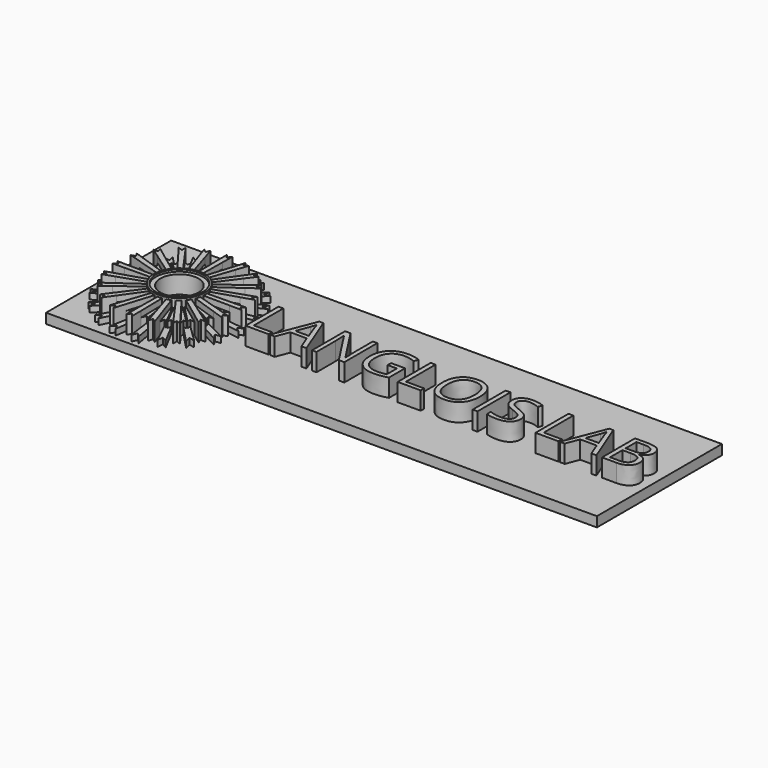
from build123d import *

# Parameters (mm, degrees)
F0_R         = 11.7672405149
F0_R_2       = 9.5549207282
F1_DEPTH     = 9
F2_DEPTH     = 10
F3_DEPTH     = 3
F4_DEPTH     = 6
F5_DEPTH     = 9
F6_TEXT_SIZE = 28.9957211175
F7_DEPTH     = 9
F9_W         = 276.4481753111
F9_H         = 78.4506313503
F10_DEPTH    = 5


# Not quite as in the source:
# - Text() gives the source's letters only with a copy of the font that has no kerning and outlines rounded to 1/6400 em; it was checked with that copy


with BuildPart() as f1:
    # F0 (on Top) → F1 (new body)
    with BuildSketch(Plane.XY):
        Circle(F0_R)
        Circle(F0_R_2, mode=Mode.SUBTRACT)
    extrude(amount=F1_DEPTH)

    # F0 (on Top) → F2 (join)
    with BuildSketch(Plane.XY):
        with BuildLine():
            ThreePointArc((12.7135907926, -0.7743630538), (12.7312599796, -0.3873606999), (12.7371515254, 0))
            ThreePointArc((12.7371515254, 0), (12.715744973, 0.7381454891), (12.6515972691, 1.4738098661))
            ThreePointArc((12.6515972691, 1.4738098661), (12.6226522142, 1.7040187972), (12.589518622, 1.9336622889))
            ThreePointArc((12.589518622, 1.9336622889), (12.5328289853, 2.2722734447), (12.4670336703, 2.609233689))
            ThreePointArc((12.4670336703, 2.609233689), (12.4022605626, 2.901544747), (12.3306347123, 3.1922525861))
            ThreePointArc((12.3306347123, 3.1922525861), (12.0006538998, 4.268411292), (11.5769517292, 5.311235039))
            ThreePointArc((11.5769517292, 5.311235039), (11.4782848741, 5.5212322293), (11.3758092138, 5.7293973254))
            ThreePointArc((11.3758092138, 5.7293973254), (11.2172575638, 6.0339176104), (11.0505560588, 6.334053976))
            ThreePointArc((11.0505560588, 6.334053976), (10.8986240881, 6.5920423215), (10.7406701937, 6.8463883012))
            ThreePointArc((10.7406701937, 6.8463883012), (10.094288463, 7.7679063721), (9.3690734927, 8.6287595208))
            ThreePointArc((9.3690734927, 8.6287595208), (9.2103430367, 8.797988982), (9.0485563398, 8.9642990326))
            ThreePointArc((9.0485563398, 8.9642990326), (8.8036628167, 9.2049198796), (8.5523730266, 9.4388529279))
            ThreePointArc((8.5523730266, 9.4388529279), (8.3281543526, 9.637264864), (8.0993340419, 9.8303518278))
            ThreePointArc((8.0993340419, 9.8303518278), (7.1998237404, 10.5070246544), (6.2440850646, 11.1016409006))
            ThreePointArc((6.2440850646, 11.1016409006), (6.0408286506, 11.213537274), (5.8355677263, 11.3217126925))
            ThreePointArc((5.8355677263, 11.3217126925), (5.5283042144, 11.4748804566), (5.2170241346, 11.6197111909))
            ThreePointArc((5.2170241346, 11.6197111909), (4.9424668435, 11.739124775), (4.6651786428, 11.8520520254))
            ThreePointArc((4.6651786428, 11.8520520254), (3.600590106, 12.2176421567), (2.5078820852, 12.4878163194))
            ThreePointArc((2.5078820852, 12.4878163194), (2.2799958672, 12.5314264083), (2.051353085, 12.5708782311))
            ThreePointArc((2.051353085, 12.5708782311), (1.7117966777, 12.6215997843), (1.3709965711, 12.6631511632))
            ThreePointArc((1.3709965711, 12.6631511632), (1.0729762435, 12.6918773616), (0.7743630538, 12.7135907926))
            ThreePointArc((0.7743630538, 12.7135907926), (-0.3510943748, 12.7323117194), (-1.4738098661, 12.6515972691))
            ThreePointArc((-1.4738098661, 12.6515972691), (-1.7040187972, 12.6226522142), (-1.9336622889, 12.589518622))
            ThreePointArc((-1.9336622889, 12.589518622), (-2.2722734447, 12.5328289853), (-2.609233689, 12.4670336703))
            ThreePointArc((-2.609233689, 12.4670336703), (-2.901544747, 12.4022605626), (-3.1922525861, 12.3306347123))
            ThreePointArc((-3.1922525861, 12.3306347123), (-4.268411292, 12.0006538998), (-5.311235039, 11.5769517292))
            ThreePointArc((-5.311235039, 11.5769517292), (-5.5212322293, 11.4782848741), (-5.7293973254, 11.3758092138))
            ThreePointArc((-5.7293973254, 11.3758092138), (-6.0339176104, 11.2172575638), (-6.334053976, 11.0505560588))
            ThreePointArc((-6.334053976, 11.0505560588), (-6.5920423215, 10.8986240881), (-6.8463883012, 10.7406701937))
            ThreePointArc((-6.8463883012, 10.7406701937), (-7.7679063721, 10.094288463), (-8.6287595208, 9.3690734927))
            ThreePointArc((-8.6287595208, 9.3690734927), (-8.797988982, 9.2103430367), (-8.9642990326, 9.0485563398))
            ThreePointArc((-8.9642990326, 9.0485563398), (-9.2049198796, 8.8036628167), (-9.4388529279, 8.5523730266))
            ThreePointArc((-9.4388529279, 8.5523730266), (-9.637264864, 8.3281543526), (-9.8303518278, 8.0993340419))
            ThreePointArc((-9.8303518278, 8.0993340419), (-10.5070246544, 7.1998237404), (-11.1016409006, 6.2440850646))
            ThreePointArc((-11.1016409006, 6.2440850646), (-11.213537274, 6.0408286506), (-11.3217126925, 5.8355677263))
            ThreePointArc((-11.3217126925, 5.8355677263), (-11.4748804566, 5.5283042144), (-11.6197111909, 5.2170241346))
            ThreePointArc((-11.6197111909, 5.2170241346), (-11.739124775, 4.9424668435), (-11.8520520254, 4.6651786428))
            ThreePointArc((-11.8520520254, 4.6651786428), (-12.2176421567, 3.600590106), (-12.4878163194, 2.5078820852))
            ThreePointArc((-12.4878163194, 2.5078820852), (-12.5314264083, 2.2799958672), (-12.5708782311, 2.051353085))
            ThreePointArc((-12.5708782311, 2.051353085), (-12.6215997843, 1.7117966777), (-12.6631511632, 1.3709965711))
            ThreePointArc((-12.6631511632, 1.3709965711), (-12.6918773616, 1.0729762435), (-12.7135907926, 0.7743630538))
            ThreePointArc((-12.7135907926, 0.7743630538), (-12.7323117194, -0.3510943748), (-12.6515972691, -1.4738098661))
            ThreePointArc((-12.6515972691, -1.4738098661), (-12.6226522142, -1.7040187972), (-12.589518622, -1.9336622889))
            ThreePointArc((-12.589518622, -1.9336622889), (-12.5328289853, -2.2722734447), (-12.4670336703, -2.609233689))
            ThreePointArc((-12.4670336703, -2.609233689), (-12.4022605626, -2.901544747), (-12.3306347123, -3.1922525861))
            ThreePointArc((-12.3306347123, -3.1922525861), (-12.0006538998, -4.268411292), (-11.5769517292, -5.311235039))
            ThreePointArc((-11.5769517292, -5.311235039), (-11.4782848741, -5.5212322293), (-11.3758092138, -5.7293973254))
            ThreePointArc((-11.3758092138, -5.7293973254), (-11.2172575638, -6.0339176104), (-11.0505560588, -6.334053976))
            ThreePointArc((-11.0505560588, -6.334053976), (-10.8986240881, -6.5920423215), (-10.7406701937, -6.8463883012))
            ThreePointArc((-10.7406701937, -6.8463883012), (-10.094288463, -7.7679063721), (-9.3690734927, -8.6287595208))
            ThreePointArc((-9.3690734927, -8.6287595208), (-9.2103430367, -8.797988982), (-9.0485563398, -8.9642990326))
            ThreePointArc((-9.0485563398, -8.9642990326), (-8.8036628167, -9.2049198796), (-8.5523730266, -9.4388529279))
            ThreePointArc((-8.5523730266, -9.4388529279), (-8.3281543526, -9.637264864), (-8.0993340419, -9.8303518278))
            ThreePointArc((-8.0993340419, -9.8303518278), (-7.1998237404, -10.5070246544), (-6.2440850646, -11.1016409006))
            ThreePointArc((-6.2440850646, -11.1016409006), (-6.0408286506, -11.213537274), (-5.8355677263, -11.3217126925))
            ThreePointArc((-5.8355677263, -11.3217126925), (-5.5283042144, -11.4748804566), (-5.2170241346, -11.6197111909))
            ThreePointArc((-5.2170241346, -11.6197111909), (-4.9424668435, -11.739124775), (-4.6651786428, -11.8520520254))
            ThreePointArc((-4.6651786428, -11.8520520254), (-3.600590106, -12.2176421567), (-2.5078820852, -12.4878163194))
            ThreePointArc((-2.5078820852, -12.4878163194), (-2.2799958672, -12.5314264083), (-2.051353085, -12.5708782311))
            ThreePointArc((-2.051353085, -12.5708782311), (-1.7117966777, -12.6215997843), (-1.3709965711, -12.6631511632))
            ThreePointArc((-1.3709965711, -12.6631511632), (-1.0729762435, -12.6918773616), (-0.7743630538, -12.7135907926))
            ThreePointArc((-0.7743630538, -12.7135907926), (0.3510943748, -12.7323117194), (1.4738098661, -12.6515972691))
            ThreePointArc((1.4738098661, -12.6515972691), (1.7040187972, -12.6226522142), (1.9336622889, -12.589518622))
            ThreePointArc((1.9336622889, -12.589518622), (2.2722734447, -12.5328289853), (2.609233689, -12.4670336703))
            ThreePointArc((2.609233689, -12.4670336703), (2.901544747, -12.4022605626), (3.1922525861, -12.3306347123))
            ThreePointArc((3.1922525861, -12.3306347123), (4.268411292, -12.0006538998), (5.311235039, -11.5769517292))
            ThreePointArc((5.311235039, -11.5769517292), (5.5212322293, -11.4782848741), (5.7293973254, -11.3758092138))
            ThreePointArc((5.7293973254, -11.3758092138), (6.0339176104, -11.2172575638), (6.334053976, -11.0505560588))
            ThreePointArc((6.334053976, -11.0505560588), (6.5920423215, -10.8986240881), (6.8463883012, -10.7406701937))
            ThreePointArc((6.8463883012, -10.7406701937), (7.7679063721, -10.094288463), (8.6287595208, -9.3690734927))
            ThreePointArc((8.6287595208, -9.3690734927), (8.797988982, -9.2103430367), (8.9642990326, -9.0485563398))
            ThreePointArc((8.9642990326, -9.0485563398), (9.2049198796, -8.8036628167), (9.4388529279, -8.5523730266))
            ThreePointArc((9.4388529279, -8.5523730266), (9.637264864, -8.3281543526), (9.8303518278, -8.0993340419))
            ThreePointArc((9.8303518278, -8.0993340419), (10.5070246544, -7.1998237404), (11.1016409006, -6.2440850646))
            ThreePointArc((11.1016409006, -6.2440850646), (11.213537274, -6.0408286506), (11.3217126925, -5.8355677263))
            ThreePointArc((11.3217126925, -5.8355677263), (11.4748804566, -5.5283042144), (11.6197111909, -5.2170241346))
            ThreePointArc((11.6197111909, -5.2170241346), (11.739124775, -4.9424668435), (11.8520520254, -4.6651786428))
            ThreePointArc((11.8520520254, -4.6651786428), (12.2176421567, -3.600590106), (12.4878163194, -2.5078820852))
            ThreePointArc((12.4878163194, -2.5078820852), (12.5314264083, -2.2799958672), (12.5708782311, -2.051353085))
            ThreePointArc((12.5708782311, -2.051353085), (12.6215997843, -1.7117966777), (12.6631511632, -1.3709965711))
            ThreePointArc((12.6631511632, -1.3709965711), (12.6918773616, -1.0729762435), (12.7135907926, -0.7743630538))
        make_face()
        Circle(F0_R, mode=Mode.SUBTRACT)
    extrude(amount=F2_DEPTH)

    # F0 (on Top) → F3 (join)
    with BuildSketch(Plane.XY):
        with BuildLine():
            Line((11.6859453374, -21.9507384227), (6.334053976, -11.0505560588))
            ThreePointArc((6.334053976, -11.0505560588), (6.0339176104, -11.2172575638), (5.7293973254, -11.3758092138))
            Line((5.7293973254, -11.3758092138), (11.2666978089, -22.2109639059))
            Line((11.2666978089, -22.2109639059), (9.8357876585, -21.7249978341))
            Line((9.8357876585, -21.7249978341), (15.0472962032, -32.4688493698))
            Line((15.0472962032, -32.4688493698), (15.3143611387, -29.4471931073))
            Line((15.3143611387, -29.4471931073), (17.853469935, -30.9337573252))
            Line((17.853469935, -30.9337573252), (12.2699130015, -20.3598729012))
            Line((12.2699130015, -20.3598729012), (11.6859453374, -21.9507384227))
        make_face()
        with BuildLine():
            Line((17.8971456739, -17.2652371098), (9.4388529279, -8.5523730266))
            ThreePointArc((9.4388529279, -8.5523730266), (9.2049198796, -8.8036628167), (8.9642990326, -9.0485563398))
            Line((8.9642990326, -9.0485563398), (17.5788316767, -17.6422808625))
            Line((17.5788316767, -17.6422808625), (16.067783479, -17.6222752171))
            Line((16.067783479, -17.6222752171), (24.3442553498, -26.2298405236))
            Line((24.3442553498, -26.2298405236), (23.6645060607, -23.2735470415))
            Line((23.6645060607, -23.2735470415), (26.5387156335, -23.9027258591))
            Line((26.5387156335, -23.9027258591), (17.9609274443, -15.5717781567))
            Line((17.9609274443, -15.5717781567), (17.8971456739, -17.2652371098))
        make_face()
        with BuildLine():
            Line((22.3564486951, -10.8896940947), (11.6197111909, -5.2170241346))
            ThreePointArc((11.6197111909, -5.2170241346), (11.4748804566, -5.5283042144), (11.3217126925, -5.8355677263))
            Line((11.3217126925, -5.8355677263), (22.170227021, -11.3466484472))
            Line((22.170227021, -11.3466484472), (20.7269527018, -11.7945615202))
            Line((20.7269527018, -11.7945615202), (31.2582291663, -17.4232721329))
            Line((31.2582291663, -17.4232721329), (29.6982042491, -14.8217240348))
            Line((29.6982042491, -14.8217240348), (32.6261669397, -14.5319290459))
            Line((32.6261669397, -14.5319290459), (21.8938011676, -9.2594092712))
            Line((21.8938011676, -9.2594092712), (22.3564486951, -10.8896940947))
        make_face()
        with BuildLine():
            Line((24.6273467515, -3.4481919485), (12.6631511632, -1.3709965711))
            ThreePointArc((12.6631511632, -1.3709965711), (12.6215997843, -1.7117966777), (12.5708782311, -2.051353085))
            Line((12.5708782311, -2.051353085), (24.5914460754, -3.9403270252))
            Line((24.5914460754, -3.9403270252), (23.3572233809, -4.8123139642))
            Line((23.3572233809, -4.8123139642), (35.1124297231, -6.9111924707))
            Line((35.1124297231, -6.9111924707), (32.8248352861, -4.9190474107))
            Line((32.8248352861, -4.9190474107), (35.519941706, -3.7386457678))
            Line((35.519941706, -3.7386457678), (23.6835570896, -2.0406648921))
            Line((23.6835570896, -2.0406648921), (24.6273467515, -3.4481919485))
        make_face()
        with BuildLine():
            ThreePointArc((12.4670336703, 2.609233689), (12.5328289853, 2.2722734447), (12.589518622, 1.9336622889))
            Line((12.589518622, 1.9336622889), (24.6054830493, 3.8517010599))
            Line((24.6054830493, 3.8517010599), (23.7011262962, 2.640996412))
            Line((23.7011262962, 2.640996412), (35.529581016, 4.2774028636))
            Line((35.529581016, 4.2774028636), (32.7383427412, 5.4651398471))
            Line((32.7383427412, 5.4651398471), (34.9367770961, 7.4206022068))
            Line((34.9367770961, 7.4206022068), (23.1550014306, 5.3778339847))
            Line((23.1550014306, 5.3778339847), (24.487548519, 4.3308432505))
            Line((24.487548519, 4.3308432505), (12.4670336703, 2.609233689))
        make_face()
        with BuildLine():
            ThreePointArc((11.0505560588, 6.334053976), (11.2172575638, 6.0339176104), (11.3758092138, 5.7293973254))
            Line((11.3758092138, 5.7293973254), (22.2109639059, 11.2666978089))
            Line((22.2109639059, 11.2666978089), (21.7249978341, 9.8357876585))
            Line((21.7249978341, 9.8357876585), (32.4688493698, 15.0472962032))
            Line((32.4688493698, 15.0472962032), (29.4471931073, 15.3143611387))
            Line((29.4471931073, 15.3143611387), (30.9337573252, 17.853469935))
            Line((30.9337573252, 17.853469935), (20.3598729012, 12.2699130015))
            Line((20.3598729012, 12.2699130015), (21.9507384227, 11.6859453374))
            Line((21.9507384227, 11.6859453374), (11.0505560588, 6.334053976))
        make_face()
        with BuildLine():
            ThreePointArc((8.5523730266, 9.4388529279), (8.8036628167, 9.2049198796), (9.0485563398, 8.9642990326))
            Line((9.0485563398, 8.9642990326), (17.6422808625, 17.5788316767))
            Line((17.6422808625, 17.5788316767), (17.6222752171, 16.067783479))
            Line((17.6222752171, 16.067783479), (26.2298405236, 24.3442553498))
            Line((26.2298405236, 24.3442553498), (23.2735470415, 23.6645060607))
            Line((23.2735470415, 23.6645060607), (23.9027258591, 26.5387156335))
            Line((23.9027258591, 26.5387156335), (15.5717781567, 17.9609274443))
            Line((15.5717781567, 17.9609274443), (17.2652371098, 17.8971456739))
            Line((17.2652371098, 17.8971456739), (8.5523730266, 9.4388529279))
        make_face()
        with BuildLine():
            ThreePointArc((5.2170241346, 11.6197111909), (5.5283042144, 11.4748804566), (5.8355677263, 11.3217126925))
            Line((5.8355677263, 11.3217126925), (11.3466484472, 22.170227021))
            Line((11.3466484472, 22.170227021), (11.7945615202, 20.7269527018))
            Line((11.7945615202, 20.7269527018), (17.4232721329, 31.2582291663))
            Line((17.4232721329, 31.2582291663), (14.8217240348, 29.6982042491))
            Line((14.8217240348, 29.6982042491), (14.5319290459, 32.6261669397))
            Line((14.5319290459, 32.6261669397), (9.2594092712, 21.8938011676))
            Line((9.2594092712, 21.8938011676), (10.8896940947, 22.3564486951))
            Line((10.8896940947, 22.3564486951), (5.2170241346, 11.6197111909))
        make_face()
        with BuildLine():
            ThreePointArc((1.3709965711, 12.6631511632), (1.7117966777, 12.6215997843), (2.051353085, 12.5708782311))
            Line((2.051353085, 12.5708782311), (3.9403270252, 24.5914460754))
            Line((3.9403270252, 24.5914460754), (4.8123139642, 23.3572233809))
            Line((4.8123139642, 23.3572233809), (6.9111924707, 35.1124297231))
            Line((6.9111924707, 35.1124297231), (4.9190474107, 32.8248352861))
            Line((4.9190474107, 32.8248352861), (3.7386457678, 35.519941706))
            Line((3.7386457678, 35.519941706), (2.0406648921, 23.6835570896))
            Line((2.0406648921, 23.6835570896), (3.4481919485, 24.6273467515))
            Line((3.4481919485, 24.6273467515), (1.3709965711, 12.6631511632))
        make_face()
        with BuildLine():
            ThreePointArc((-2.609233689, 12.4670336703), (-2.2722734447, 12.5328289853), (-1.9336622889, 12.589518622))
            Line((-1.9336622889, 12.589518622), (-3.8517010599, 24.6054830493))
            Line((-3.8517010599, 24.6054830493), (-2.640996412, 23.7011262962))
            Line((-2.640996412, 23.7011262962), (-4.2774028636, 35.529581016))
            Line((-4.2774028636, 35.529581016), (-5.4651398471, 32.7383427412))
            Line((-5.4651398471, 32.7383427412), (-7.4206022068, 34.9367770961))
            Line((-7.4206022068, 34.9367770961), (-5.3778339847, 23.1550014306))
            Line((-5.3778339847, 23.1550014306), (-4.3308432505, 24.487548519))
            Line((-4.3308432505, 24.487548519), (-2.609233689, 12.4670336703))
        make_face()
        with BuildLine():
            ThreePointArc((-6.334053976, 11.0505560588), (-6.0339176104, 11.2172575638), (-5.7293973254, 11.3758092138))
            Line((-5.7293973254, 11.3758092138), (-11.2666978089, 22.2109639059))
            Line((-11.2666978089, 22.2109639059), (-9.8357876585, 21.7249978341))
            Line((-9.8357876585, 21.7249978341), (-15.0472962032, 32.4688493698))
            Line((-15.0472962032, 32.4688493698), (-15.3143611387, 29.4471931073))
            Line((-15.3143611387, 29.4471931073), (-17.853469935, 30.9337573252))
            Line((-17.853469935, 30.9337573252), (-12.2699130015, 20.3598729012))
            Line((-12.2699130015, 20.3598729012), (-11.6859453374, 21.9507384227))
            Line((-11.6859453374, 21.9507384227), (-6.334053976, 11.0505560588))
        make_face()
        with BuildLine():
            ThreePointArc((-9.4388529279, 8.5523730266), (-9.2049198796, 8.8036628167), (-8.9642990326, 9.0485563398))
            Line((-8.9642990326, 9.0485563398), (-17.5788316767, 17.6422808625))
            Line((-17.5788316767, 17.6422808625), (-16.067783479, 17.6222752171))
            Line((-16.067783479, 17.6222752171), (-24.3442553498, 26.2298405236))
            Line((-24.3442553498, 26.2298405236), (-23.6645060607, 23.2735470415))
            Line((-23.6645060607, 23.2735470415), (-26.5387156335, 23.9027258591))
            Line((-26.5387156335, 23.9027258591), (-17.9609274443, 15.5717781567))
            Line((-17.9609274443, 15.5717781567), (-17.8971456739, 17.2652371098))
            Line((-17.8971456739, 17.2652371098), (-9.4388529279, 8.5523730266))
        make_face()
        with BuildLine():
            ThreePointArc((-11.6197111909, 5.2170241346), (-11.4748804566, 5.5283042144), (-11.3217126925, 5.8355677263))
            Line((-11.3217126925, 5.8355677263), (-22.170227021, 11.3466484472))
            Line((-22.170227021, 11.3466484472), (-20.7269527018, 11.7945615202))
            Line((-20.7269527018, 11.7945615202), (-31.2582291663, 17.4232721329))
            Line((-31.2582291663, 17.4232721329), (-29.6982042491, 14.8217240348))
            Line((-29.6982042491, 14.8217240348), (-32.6261669397, 14.5319290459))
            Line((-32.6261669397, 14.5319290459), (-21.8938011676, 9.2594092712))
            Line((-21.8938011676, 9.2594092712), (-22.3564486951, 10.8896940947))
            Line((-22.3564486951, 10.8896940947), (-11.6197111909, 5.2170241346))
        make_face()
        with BuildLine():
            ThreePointArc((-12.6631511632, 1.3709965711), (-12.6215997843, 1.7117966777), (-12.5708782311, 2.051353085))
            Line((-12.5708782311, 2.051353085), (-24.5914460754, 3.9403270252))
            Line((-24.5914460754, 3.9403270252), (-23.3572233809, 4.8123139642))
            Line((-23.3572233809, 4.8123139642), (-35.1124297231, 6.9111924707))
            Line((-35.1124297231, 6.9111924707), (-32.8248352861, 4.9190474107))
            Line((-32.8248352861, 4.9190474107), (-35.519941706, 3.7386457678))
            Line((-35.519941706, 3.7386457678), (-23.6835570896, 2.0406648921))
            Line((-23.6835570896, 2.0406648921), (-24.6273467515, 3.4481919485))
            Line((-24.6273467515, 3.4481919485), (-12.6631511632, 1.3709965711))
        make_face()
        with BuildLine():
            Line((-24.487548519, -4.3308432505), (-12.4670336703, -2.609233689))
            ThreePointArc((-12.4670336703, -2.609233689), (-12.5328289853, -2.2722734447), (-12.589518622, -1.9336622889))
            Line((-12.589518622, -1.9336622889), (-24.6054830493, -3.8517010599))
            Line((-24.6054830493, -3.8517010599), (-23.7011262962, -2.640996412))
            Line((-23.7011262962, -2.640996412), (-35.529581016, -4.2774028636))
            Line((-35.529581016, -4.2774028636), (-32.7383427412, -5.4651398471))
            Line((-32.7383427412, -5.4651398471), (-34.9367770961, -7.4206022068))
            Line((-34.9367770961, -7.4206022068), (-23.1550014306, -5.3778339847))
            Line((-23.1550014306, -5.3778339847), (-24.487548519, -4.3308432505))
        make_face()
        with BuildLine():
            Line((-21.9507384227, -11.6859453374), (-11.0505560588, -6.334053976))
            ThreePointArc((-11.0505560588, -6.334053976), (-11.2172575638, -6.0339176104), (-11.3758092138, -5.7293973254))
            Line((-11.3758092138, -5.7293973254), (-22.2109639059, -11.2666978089))
            Line((-22.2109639059, -11.2666978089), (-21.7249978341, -9.8357876585))
            Line((-21.7249978341, -9.8357876585), (-32.4688493698, -15.0472962032))
            Line((-32.4688493698, -15.0472962032), (-29.4471931073, -15.3143611387))
            Line((-29.4471931073, -15.3143611387), (-30.9337573252, -17.853469935))
            Line((-30.9337573252, -17.853469935), (-20.3598729012, -12.2699130015))
            Line((-20.3598729012, -12.2699130015), (-21.9507384227, -11.6859453374))
        make_face()
        with BuildLine():
            Line((-17.2652371098, -17.8971456739), (-8.5523730266, -9.4388529279))
            ThreePointArc((-8.5523730266, -9.4388529279), (-8.8036628167, -9.2049198796), (-9.0485563398, -8.9642990326))
            Line((-9.0485563398, -8.9642990326), (-17.6422808625, -17.5788316767))
            Line((-17.6422808625, -17.5788316767), (-17.6222752171, -16.067783479))
            Line((-17.6222752171, -16.067783479), (-26.2298405236, -24.3442553498))
            Line((-26.2298405236, -24.3442553498), (-23.2735470415, -23.6645060607))
            Line((-23.2735470415, -23.6645060607), (-23.9027258591, -26.5387156335))
            Line((-23.9027258591, -26.5387156335), (-15.5717781567, -17.9609274443))
            Line((-15.5717781567, -17.9609274443), (-17.2652371098, -17.8971456739))
        make_face()
        with BuildLine():
            Line((-10.8896940947, -22.3564486951), (-5.2170241346, -11.6197111909))
            ThreePointArc((-5.2170241346, -11.6197111909), (-5.5283042144, -11.4748804566), (-5.8355677263, -11.3217126925))
            Line((-5.8355677263, -11.3217126925), (-11.3466484472, -22.170227021))
            Line((-11.3466484472, -22.170227021), (-11.7945615202, -20.7269527018))
            Line((-11.7945615202, -20.7269527018), (-17.4232721329, -31.2582291663))
            Line((-17.4232721329, -31.2582291663), (-14.8217240348, -29.6982042491))
            Line((-14.8217240348, -29.6982042491), (-14.5319290459, -32.6261669397))
            Line((-14.5319290459, -32.6261669397), (-9.2594092712, -21.8938011676))
            Line((-9.2594092712, -21.8938011676), (-10.8896940947, -22.3564486951))
        make_face()
        with BuildLine():
            Line((-3.4481919485, -24.6273467515), (-1.3709965711, -12.6631511632))
            ThreePointArc((-1.3709965711, -12.6631511632), (-1.7117966777, -12.6215997843), (-2.051353085, -12.5708782311))
            Line((-2.051353085, -12.5708782311), (-3.9403270252, -24.5914460754))
            Line((-3.9403270252, -24.5914460754), (-4.8123139642, -23.3572233809))
            Line((-4.8123139642, -23.3572233809), (-6.9111924707, -35.1124297231))
            Line((-6.9111924707, -35.1124297231), (-4.9190474107, -32.8248352861))
            Line((-4.9190474107, -32.8248352861), (-3.7386457678, -35.519941706))
            Line((-3.7386457678, -35.519941706), (-2.0406648921, -23.6835570896))
            Line((-2.0406648921, -23.6835570896), (-3.4481919485, -24.6273467515))
        make_face()
        with BuildLine():
            Line((4.3308432505, -24.487548519), (2.609233689, -12.4670336703))
            ThreePointArc((2.609233689, -12.4670336703), (2.2722734447, -12.5328289853), (1.9336622889, -12.589518622))
            Line((1.9336622889, -12.589518622), (3.8517010599, -24.6054830493))
            Line((3.8517010599, -24.6054830493), (2.640996412, -23.7011262962))
            Line((2.640996412, -23.7011262962), (4.2774028636, -35.529581016))
            Line((4.2774028636, -35.529581016), (5.4651398471, -32.7383427412))
            Line((5.4651398471, -32.7383427412), (7.4206022068, -34.9367770961))
            Line((7.4206022068, -34.9367770961), (5.3778339847, -23.1550014306))
            Line((5.3778339847, -23.1550014306), (4.3308432505, -24.487548519))
        make_face()
    extrude(amount=F3_DEPTH)

    # F0 (on Top) → F4 (join)
    with BuildSketch(Plane.XY):
        with BuildLine():
            Line((-17.6422808625, -17.5788316767), (-9.0485563398, -8.9642990326))
            ThreePointArc((-9.0485563398, -8.9642990326), (-9.2103430367, -8.797988982), (-9.3690734927, -8.6287595208))
            Line((-9.3690734927, -8.6287595208), (-20.1457536449, -16.6949031094))
            Line((-20.1457536449, -16.6949031094), (-17.6222752171, -16.067783479))
            Line((-17.6222752171, -16.067783479), (-17.6422808625, -17.5788316767))
        make_face()
        with BuildLine():
            Line((-15.9299640597, -20.3504452441), (-8.0993340419, -9.8303518278))
            ThreePointArc((-8.0993340419, -9.8303518278), (-8.3281543526, -9.637264864), (-8.5523730266, -9.4388529279))
            Line((-8.5523730266, -9.4388529279), (-17.2652371098, -17.8971456739))
            Line((-17.2652371098, -17.8971456739), (-15.5717781567, -17.9609274443))
            Line((-15.5717781567, -17.9609274443), (-15.9299640597, -20.3504452441))
        make_face()
        with BuildLine():
            Line((-11.3466484472, -22.170227021), (-5.8355677263, -11.3217126925))
            ThreePointArc((-5.8355677263, -11.3217126925), (-6.0408286506, -11.213537274), (-6.2440850646, -11.1016409006))
            Line((-6.2440850646, -11.1016409006), (-14.0007414995, -22.1031766319))
            Line((-14.0007414995, -22.1031766319), (-11.7945615202, -20.7269527018))
            Line((-11.7945615202, -20.7269527018), (-11.3466484472, -22.170227021))
        make_face()
        with BuildLine():
            Line((-8.8616626998, -24.2770531732), (-4.6651786428, -11.8520520254))
            ThreePointArc((-4.6651786428, -11.8520520254), (-4.9424668435, -11.739124775), (-5.2170241346, -11.6197111909))
            Line((-5.2170241346, -11.6197111909), (-10.8896940947, -22.3564486951))
            Line((-10.8896940947, -22.3564486951), (-9.2594092712, -21.8938011676))
            Line((-9.2594092712, -21.8938011676), (-8.8616626998, -24.2770531732))
        make_face()
        with BuildLine():
            Line((-3.9403270252, -24.5914460754), (-2.051353085, -12.5708782311))
            ThreePointArc((-2.051353085, -12.5708782311), (-2.2799958672, -12.5314264083), (-2.5078820852, -12.4878163194))
            Line((-2.5078820852, -12.4878163194), (-6.4852392271, -25.3478372238))
            Line((-6.4852392271, -25.3478372238), (-4.8123139642, -23.3572233809))
            Line((-4.8123139642, -23.3572233809), (-3.9403270252, -24.5914460754))
        make_face()
        with BuildLine():
            Line((-0.925920052, -25.8272539894), (-0.7743630538, -12.7135907926))
            ThreePointArc((-0.7743630538, -12.7135907926), (-1.0729762435, -12.6918773616), (-1.3709965711, -12.6631511632))
            Line((-1.3709965711, -12.6631511632), (-3.4481919485, -24.6273467515))
            Line((-3.4481919485, -24.6273467515), (-2.0406648921, -23.6835570896))
            Line((-2.0406648921, -23.6835570896), (-0.925920052, -25.8272539894))
        make_face()
        with BuildLine():
            Line((3.8517010599, -24.6054830493), (1.9336622889, -12.589518622))
            ThreePointArc((1.9336622889, -12.589518622), (1.7040187972, -12.6226522142), (1.4738098661, -12.6515972691))
            Line((1.4738098661, -12.6515972691), (1.6650834461, -26.1112748994))
            Line((1.6650834461, -26.1112748994), (2.640996412, -23.7011262962))
            Line((2.640996412, -23.7011262962), (3.8517010599, -24.6054830493))
        make_face()
        with BuildLine():
            Line((7.1004581018, -24.8493032362), (3.1922525861, -12.3306347123))
            ThreePointArc((3.1922525861, -12.3306347123), (2.901544747, -12.4022605626), (2.609233689, -12.4670336703))
            Line((2.609233689, -12.4670336703), (4.3308432505, -24.487548519))
            Line((4.3308432505, -24.487548519), (5.3778339847, -23.1550014306))
            Line((5.3778339847, -23.1550014306), (7.1004581018, -24.8493032362))
        make_face()
        with BuildLine():
            Line((11.2666978089, -22.2109639059), (5.7293973254, -11.3758092138))
            ThreePointArc((5.7293973254, -11.3758092138), (5.5212322293, -11.4782848741), (5.311235039, -11.5769517292))
            Line((5.311235039, -11.5769517292), (9.6524161503, -24.31875906))
            Line((9.6524161503, -24.31875906), (9.8357876585, -21.7249978341))
            Line((9.8357876585, -21.7249978341), (11.2666978089, -22.2109639059))
        make_face()
        with BuildLine():
            Line((14.4317939447, -21.4389295469), (6.8463883012, -10.7406701937))
            ThreePointArc((6.8463883012, -10.7406701937), (6.5920423215, -10.8986240881), (6.334053976, -11.0505560588))
            Line((6.334053976, -11.0505560588), (11.6859453374, -21.9507384227))
            Line((11.6859453374, -21.9507384227), (12.2699130015, -20.3598729012))
            Line((12.2699130015, -20.3598729012), (14.4317939447, -21.4389295469))
        make_face()
        with BuildLine():
            Line((17.5788316767, -17.6422808625), (8.9642990326, -9.0485563398))
            ThreePointArc((8.9642990326, -9.0485563398), (8.797988982, -9.2103430367), (8.6287595208, -9.3690734927))
            Line((8.6287595208, -9.3690734927), (16.6949031094, -20.1457536449))
            Line((16.6949031094, -20.1457536449), (16.067783479, -17.6222752171))
            Line((16.067783479, -17.6222752171), (17.5788316767, -17.6422808625))
        make_face()
        with BuildLine():
            Line((20.3504452441, -15.9299640597), (9.8303518278, -8.0993340419))
            ThreePointArc((9.8303518278, -8.0993340419), (9.637264864, -8.3281543526), (9.4388529279, -8.5523730266))
            Line((9.4388529279, -8.5523730266), (17.8971456739, -17.2652371098))
            Line((17.8971456739, -17.2652371098), (17.9609274443, -15.5717781567))
            Line((17.9609274443, -15.5717781567), (20.3504452441, -15.9299640597))
        make_face()
        with BuildLine():
            Line((22.170227021, -11.3466484472), (11.3217126925, -5.8355677263))
            ThreePointArc((11.3217126925, -5.8355677263), (11.213537274, -6.0408286506), (11.1016409006, -6.2440850646))
            Line((11.1016409006, -6.2440850646), (22.1031766319, -14.0007414995))
            Line((22.1031766319, -14.0007414995), (20.7269527018, -11.7945615202))
            Line((20.7269527018, -11.7945615202), (22.170227021, -11.3466484472))
        make_face()
        with BuildLine():
            Line((24.2770531732, -8.8616626998), (11.8520520254, -4.6651786428))
            ThreePointArc((11.8520520254, -4.6651786428), (11.739124775, -4.9424668435), (11.6197111909, -5.2170241346))
            Line((11.6197111909, -5.2170241346), (22.3564486951, -10.8896940947))
            Line((22.3564486951, -10.8896940947), (21.8938011676, -9.2594092712))
            Line((21.8938011676, -9.2594092712), (24.2770531732, -8.8616626998))
        make_face()
        with BuildLine():
            Line((24.5914460754, -3.9403270252), (12.5708782311, -2.051353085))
            ThreePointArc((12.5708782311, -2.051353085), (12.5314264083, -2.2799958672), (12.4878163194, -2.5078820852))
            Line((12.4878163194, -2.5078820852), (25.3478372238, -6.4852392271))
            Line((25.3478372238, -6.4852392271), (23.3572233809, -4.8123139642))
            Line((23.3572233809, -4.8123139642), (24.5914460754, -3.9403270252))
        make_face()
        with BuildLine():
            Line((25.8272539894, -0.925920052), (12.7135907926, -0.7743630538))
            ThreePointArc((12.7135907926, -0.7743630538), (12.6918773616, -1.0729762435), (12.6631511632, -1.3709965711))
            Line((12.6631511632, -1.3709965711), (24.6273467515, -3.4481919485))
            Line((24.6273467515, -3.4481919485), (23.6835570896, -2.0406648921))
            Line((23.6835570896, -2.0406648921), (25.8272539894, -0.925920052))
        make_face()
        with BuildLine():
            ThreePointArc((12.589518622, 1.9336622889), (12.6226522142, 1.7040187972), (12.6515972691, 1.4738098661))
            Line((12.6515972691, 1.4738098661), (26.1112748994, 1.6650834461))
            Line((26.1112748994, 1.6650834461), (23.7011262962, 2.640996412))
            Line((23.7011262962, 2.640996412), (24.6054830493, 3.8517010599))
            Line((24.6054830493, 3.8517010599), (12.589518622, 1.9336622889))
        make_face()
        with BuildLine():
            ThreePointArc((12.3306347123, 3.1922525861), (12.4022605626, 2.901544747), (12.4670336703, 2.609233689))
            Line((12.4670336703, 2.609233689), (24.487548519, 4.3308432505))
            Line((24.487548519, 4.3308432505), (23.1550014306, 5.3778339847))
            Line((23.1550014306, 5.3778339847), (24.8493032362, 7.1004581018))
            Line((24.8493032362, 7.1004581018), (12.3306347123, 3.1922525861))
        make_face()
        with BuildLine():
            ThreePointArc((11.3758092138, 5.7293973254), (11.4782848741, 5.5212322293), (11.5769517292, 5.311235039))
            Line((11.5769517292, 5.311235039), (24.31875906, 9.6524161503))
            Line((24.31875906, 9.6524161503), (21.7249978341, 9.8357876585))
            Line((21.7249978341, 9.8357876585), (22.2109639059, 11.2666978089))
            Line((22.2109639059, 11.2666978089), (11.3758092138, 5.7293973254))
        make_face()
        with BuildLine():
            ThreePointArc((10.7406701937, 6.8463883012), (10.8986240881, 6.5920423215), (11.0505560588, 6.334053976))
            Line((11.0505560588, 6.334053976), (21.9507384227, 11.6859453374))
            Line((21.9507384227, 11.6859453374), (20.3598729012, 12.2699130015))
            Line((20.3598729012, 12.2699130015), (21.4389295469, 14.4317939447))
            Line((21.4389295469, 14.4317939447), (10.7406701937, 6.8463883012))
        make_face()
        with BuildLine():
            ThreePointArc((9.0485563398, 8.9642990326), (9.2103430367, 8.797988982), (9.3690734927, 8.6287595208))
            Line((9.3690734927, 8.6287595208), (20.1457536449, 16.6949031094))
            Line((20.1457536449, 16.6949031094), (17.6222752171, 16.067783479))
            Line((17.6222752171, 16.067783479), (17.6422808625, 17.5788316767))
            Line((17.6422808625, 17.5788316767), (9.0485563398, 8.9642990326))
        make_face()
        with BuildLine():
            ThreePointArc((8.0993340419, 9.8303518278), (8.3281543526, 9.637264864), (8.5523730266, 9.4388529279))
            Line((8.5523730266, 9.4388529279), (17.2652371098, 17.8971456739))
            Line((17.2652371098, 17.8971456739), (15.5717781567, 17.9609274443))
            Line((15.5717781567, 17.9609274443), (15.9299640597, 20.3504452441))
            Line((15.9299640597, 20.3504452441), (8.0993340419, 9.8303518278))
        make_face()
        with BuildLine():
            ThreePointArc((5.8355677263, 11.3217126925), (6.0408286506, 11.213537274), (6.2440850646, 11.1016409006))
            Line((6.2440850646, 11.1016409006), (14.0007414995, 22.1031766319))
            Line((14.0007414995, 22.1031766319), (11.7945615202, 20.7269527018))
            Line((11.7945615202, 20.7269527018), (11.3466484472, 22.170227021))
            Line((11.3466484472, 22.170227021), (5.8355677263, 11.3217126925))
        make_face()
        with BuildLine():
            ThreePointArc((4.6651786428, 11.8520520254), (4.9424668435, 11.739124775), (5.2170241346, 11.6197111909))
            Line((5.2170241346, 11.6197111909), (10.8896940947, 22.3564486951))
            Line((10.8896940947, 22.3564486951), (9.2594092712, 21.8938011676))
            Line((9.2594092712, 21.8938011676), (8.8616626998, 24.2770531732))
            Line((8.8616626998, 24.2770531732), (4.6651786428, 11.8520520254))
        make_face()
        with BuildLine():
            ThreePointArc((2.051353085, 12.5708782311), (2.2799958672, 12.5314264083), (2.5078820852, 12.4878163194))
            Line((2.5078820852, 12.4878163194), (6.4852392271, 25.3478372238))
            Line((6.4852392271, 25.3478372238), (4.8123139642, 23.3572233809))
            Line((4.8123139642, 23.3572233809), (3.9403270252, 24.5914460754))
            Line((3.9403270252, 24.5914460754), (2.051353085, 12.5708782311))
        make_face()
        with BuildLine():
            ThreePointArc((0.7743630538, 12.7135907926), (1.0729762435, 12.6918773616), (1.3709965711, 12.6631511632))
            Line((1.3709965711, 12.6631511632), (3.4481919485, 24.6273467515))
            Line((3.4481919485, 24.6273467515), (2.0406648921, 23.6835570896))
            Line((2.0406648921, 23.6835570896), (0.925920052, 25.8272539894))
            Line((0.925920052, 25.8272539894), (0.7743630538, 12.7135907926))
        make_face()
        with BuildLine():
            ThreePointArc((-1.9336622889, 12.589518622), (-1.7040187972, 12.6226522142), (-1.4738098661, 12.6515972691))
            Line((-1.4738098661, 12.6515972691), (-1.6650834461, 26.1112748994))
            Line((-1.6650834461, 26.1112748994), (-2.640996412, 23.7011262962))
            Line((-2.640996412, 23.7011262962), (-3.8517010599, 24.6054830493))
            Line((-3.8517010599, 24.6054830493), (-1.9336622889, 12.589518622))
        make_face()
        with BuildLine():
            ThreePointArc((-3.1922525861, 12.3306347123), (-2.901544747, 12.4022605626), (-2.609233689, 12.4670336703))
            Line((-2.609233689, 12.4670336703), (-4.3308432505, 24.487548519))
            Line((-4.3308432505, 24.487548519), (-5.3778339847, 23.1550014306))
            Line((-5.3778339847, 23.1550014306), (-7.1004581018, 24.8493032362))
            Line((-7.1004581018, 24.8493032362), (-3.1922525861, 12.3306347123))
        make_face()
        with BuildLine():
            ThreePointArc((-5.7293973254, 11.3758092138), (-5.5212322293, 11.4782848741), (-5.311235039, 11.5769517292))
            Line((-5.311235039, 11.5769517292), (-9.6524161503, 24.31875906))
            Line((-9.6524161503, 24.31875906), (-9.8357876585, 21.7249978341))
            Line((-9.8357876585, 21.7249978341), (-11.2666978089, 22.2109639059))
            Line((-11.2666978089, 22.2109639059), (-5.7293973254, 11.3758092138))
        make_face()
        with BuildLine():
            ThreePointArc((-6.8463883012, 10.7406701937), (-6.5920423215, 10.8986240881), (-6.334053976, 11.0505560588))
            Line((-6.334053976, 11.0505560588), (-11.6859453374, 21.9507384227))
            Line((-11.6859453374, 21.9507384227), (-12.2699130015, 20.3598729012))
            Line((-12.2699130015, 20.3598729012), (-14.4317939447, 21.4389295469))
            Line((-14.4317939447, 21.4389295469), (-6.8463883012, 10.7406701937))
        make_face()
        with BuildLine():
            ThreePointArc((-8.9642990326, 9.0485563398), (-8.797988982, 9.2103430367), (-8.6287595208, 9.3690734927))
            Line((-8.6287595208, 9.3690734927), (-16.6949031094, 20.1457536449))
            Line((-16.6949031094, 20.1457536449), (-16.067783479, 17.6222752171))
            Line((-16.067783479, 17.6222752171), (-17.5788316767, 17.6422808625))
            Line((-17.5788316767, 17.6422808625), (-8.9642990326, 9.0485563398))
        make_face()
        with BuildLine():
            ThreePointArc((-9.8303518278, 8.0993340419), (-9.637264864, 8.3281543526), (-9.4388529279, 8.5523730266))
            Line((-9.4388529279, 8.5523730266), (-17.8971456739, 17.2652371098))
            Line((-17.8971456739, 17.2652371098), (-17.9609274443, 15.5717781567))
            Line((-17.9609274443, 15.5717781567), (-20.3504452441, 15.9299640597))
            Line((-20.3504452441, 15.9299640597), (-9.8303518278, 8.0993340419))
        make_face()
        with BuildLine():
            ThreePointArc((-11.3217126925, 5.8355677263), (-11.213537274, 6.0408286506), (-11.1016409006, 6.2440850646))
            Line((-11.1016409006, 6.2440850646), (-22.1031766319, 14.0007414995))
            Line((-22.1031766319, 14.0007414995), (-20.7269527018, 11.7945615202))
            Line((-20.7269527018, 11.7945615202), (-22.170227021, 11.3466484472))
            Line((-22.170227021, 11.3466484472), (-11.3217126925, 5.8355677263))
        make_face()
        with BuildLine():
            ThreePointArc((-11.8520520254, 4.6651786428), (-11.739124775, 4.9424668435), (-11.6197111909, 5.2170241346))
            Line((-11.6197111909, 5.2170241346), (-22.3564486951, 10.8896940947))
            Line((-22.3564486951, 10.8896940947), (-21.8938011676, 9.2594092712))
            Line((-21.8938011676, 9.2594092712), (-24.2770531732, 8.8616626998))
            Line((-24.2770531732, 8.8616626998), (-11.8520520254, 4.6651786428))
        make_face()
        with BuildLine():
            ThreePointArc((-12.5708782311, 2.051353085), (-12.5314264083, 2.2799958672), (-12.4878163194, 2.5078820852))
            Line((-12.4878163194, 2.5078820852), (-25.3478372238, 6.4852392271))
            Line((-25.3478372238, 6.4852392271), (-23.3572233809, 4.8123139642))
            Line((-23.3572233809, 4.8123139642), (-24.5914460754, 3.9403270252))
            Line((-24.5914460754, 3.9403270252), (-12.5708782311, 2.051353085))
        make_face()
        with BuildLine():
            ThreePointArc((-12.7135907926, 0.7743630538), (-12.6918773616, 1.0729762435), (-12.6631511632, 1.3709965711))
            Line((-12.6631511632, 1.3709965711), (-24.6273467515, 3.4481919485))
            Line((-24.6273467515, 3.4481919485), (-23.6835570896, 2.0406648921))
            Line((-23.6835570896, 2.0406648921), (-25.8272539894, 0.925920052))
            Line((-25.8272539894, 0.925920052), (-12.7135907926, 0.7743630538))
        make_face()
        with BuildLine():
            Line((-24.6054830493, -3.8517010599), (-12.589518622, -1.9336622889))
            ThreePointArc((-12.589518622, -1.9336622889), (-12.6226522142, -1.7040187972), (-12.6515972691, -1.4738098661))
            Line((-12.6515972691, -1.4738098661), (-26.1112748994, -1.6650834461))
            Line((-26.1112748994, -1.6650834461), (-23.7011262962, -2.640996412))
            Line((-23.7011262962, -2.640996412), (-24.6054830493, -3.8517010599))
        make_face()
        with BuildLine():
            Line((-24.8493032362, -7.1004581018), (-12.3306347123, -3.1922525861))
            ThreePointArc((-12.3306347123, -3.1922525861), (-12.4022605626, -2.901544747), (-12.4670336703, -2.609233689))
            Line((-12.4670336703, -2.609233689), (-24.487548519, -4.3308432505))
            Line((-24.487548519, -4.3308432505), (-23.1550014306, -5.3778339847))
            Line((-23.1550014306, -5.3778339847), (-24.8493032362, -7.1004581018))
        make_face()
        with BuildLine():
            Line((-22.2109639059, -11.2666978089), (-11.3758092138, -5.7293973254))
            ThreePointArc((-11.3758092138, -5.7293973254), (-11.4782848741, -5.5212322293), (-11.5769517292, -5.311235039))
            Line((-11.5769517292, -5.311235039), (-24.31875906, -9.6524161503))
            Line((-24.31875906, -9.6524161503), (-21.7249978341, -9.8357876585))
            Line((-21.7249978341, -9.8357876585), (-22.2109639059, -11.2666978089))
        make_face()
        with BuildLine():
            Line((-21.4389295469, -14.4317939447), (-10.7406701937, -6.8463883012))
            ThreePointArc((-10.7406701937, -6.8463883012), (-10.8986240881, -6.5920423215), (-11.0505560588, -6.334053976))
            Line((-11.0505560588, -6.334053976), (-21.9507384227, -11.6859453374))
            Line((-21.9507384227, -11.6859453374), (-20.3598729012, -12.2699130015))
            Line((-20.3598729012, -12.2699130015), (-21.4389295469, -14.4317939447))
        make_face()
    extrude(amount=F4_DEPTH)

    # F0 (on Top) → F5 (join)
    with BuildSketch(Plane.XY):
        with BuildLine():
            Line((-6.4852392271, -25.3478372238), (-2.5078820852, -12.4878163194))
            ThreePointArc((-2.5078820852, -12.4878163194), (-3.600590106, -12.2176421567), (-4.6651786428, -11.8520520254))
            Line((-4.6651786428, -11.8520520254), (-8.8616626998, -24.2770531732))
            Line((-8.8616626998, -24.2770531732), (-10.8272434383, -30.0967685826))
            Line((-10.8272434383, -30.0967685826), (-8.9481921765, -28.8431892633))
            Line((-8.9481921765, -28.8431892633), (-8.2401998564, -31.0221655715))
            Line((-8.2401998564, -31.0221655715), (-6.4852392271, -25.3478372238))
        make_face()
        with BuildLine():
            Line((1.6650834461, -26.1112748994), (1.4738098661, -12.6515972691))
            ThreePointArc((1.4738098661, -12.6515972691), (0.3510943748, -12.7323117194), (-0.7743630538, -12.7135907926))
            Line((-0.7743630538, -12.7135907926), (-0.925920052, -25.8272539894))
            Line((-0.925920052, -25.8272539894), (-0.9969074577, -31.9695301046))
            Line((-0.9969074577, -31.9695301046), (0.4027991758, -30.1966465511))
            Line((0.4027991758, -30.1966465511), (1.7494805949, -32.050194509))
            Line((1.7494805949, -32.050194509), (1.6650834461, -26.1112748994))
        make_face()
        with BuildLine():
            Line((9.6524161503, -24.31875906), (5.311235039, -11.5769517292))
            ThreePointArc((5.311235039, -11.5769517292), (4.268411292, -12.0006538998), (3.1922525861, -12.3306347123))
            Line((3.1922525861, -12.3306347123), (7.1004581018, -24.8493032362))
            Line((7.1004581018, -24.8493032362), (8.9310127707, -30.7128912751))
            Line((8.9310127707, -30.7128912751), (9.7143617383, -28.594245682))
            Line((9.7143617383, -28.594245682), (11.5679096962, -29.9409271011))
            Line((11.5679096962, -29.9409271011), (9.6524161503, -24.31875906))
        make_face()
        with BuildLine():
            Line((16.6949031094, -20.1457536449), (8.6287595208, -9.3690734927))
            ThreePointArc((8.6287595208, -9.3690734927), (7.7679063721, -10.094288463), (6.8463883012, -10.7406701937))
            Line((6.8463883012, -10.7406701937), (14.4317939447, -21.4389295469))
            Line((14.4317939447, -21.4389295469), (17.9847032431, -26.4498606583))
            Line((17.9847032431, -26.4498606583), (18.0750148899, -24.1928408178))
            Line((18.0750148899, -24.1928408178), (20.2539911981, -24.9008331379))
            Line((20.2539911981, -24.9008331379), (16.6949031094, -20.1457536449))
        make_face()
        with BuildLine():
            Line((22.1031766319, -14.0007414995), (11.1016409006, -6.2440850646))
            ThreePointArc((11.1016409006, -6.2440850646), (10.5070246544, -7.1998237404), (9.8303518278, -8.0993340419))
            Line((9.8303518278, -8.0993340419), (20.3504452441, -15.9299640597))
            Line((20.3504452441, -15.9299640597), (25.2779256552, -19.5977333933))
            Line((25.2779256552, -19.5977333933), (24.6663596481, -17.4232721329))
            Line((24.6663596481, -17.4232721329), (26.9574709237, -17.4232721329))
            Line((26.9574709237, -17.4232721329), (22.1031766319, -14.0007414995))
        make_face()
        with BuildLine():
            Line((25.3478372238, -6.4852392271), (12.4878163194, -2.5078820852))
            ThreePointArc((12.4878163194, -2.5078820852), (12.2176421567, -3.600590106), (11.8520520254, -4.6651786428))
            Line((11.8520520254, -4.6651786428), (24.2770531732, -8.8616626998))
            Line((24.2770531732, -8.8616626998), (30.0967685826, -10.8272434383))
            Line((30.0967685826, -10.8272434383), (28.8431892633, -8.9481921765))
            Line((28.8431892633, -8.9481921765), (31.0221655715, -8.2401998564))
            Line((31.0221655715, -8.2401998564), (25.3478372238, -6.4852392271))
        make_face()
        with BuildLine():
            ThreePointArc((12.6515972691, 1.4738098661), (12.715744973, 0.7381454891), (12.7371515254, 0))
            ThreePointArc((12.7371515254, 0), (12.7312599796, -0.3873606999), (12.7135907926, -0.7743630538))
            Line((12.7135907926, -0.7743630538), (25.8272539894, -0.925920052))
            Line((25.8272539894, -0.925920052), (31.9695301046, -0.9969074577))
            Line((31.9695301046, -0.9969074577), (30.1966465511, 0.4027991758))
            Line((30.1966465511, 0.4027991758), (32.050194509, 1.7494805949))
            Line((32.050194509, 1.7494805949), (26.1112748994, 1.6650834461))
            Line((26.1112748994, 1.6650834461), (12.6515972691, 1.4738098661))
        make_face()
        with BuildLine():
            ThreePointArc((11.5769517292, 5.311235039), (12.0006538998, 4.268411292), (12.3306347123, 3.1922525861))
            Line((12.3306347123, 3.1922525861), (24.8493032362, 7.1004581018))
            Line((24.8493032362, 7.1004581018), (30.7128912751, 8.9310127707))
            Line((30.7128912751, 8.9310127707), (28.594245682, 9.7143617383))
            Line((28.594245682, 9.7143617383), (29.9409271011, 11.5679096962))
            Line((29.9409271011, 11.5679096962), (24.31875906, 9.6524161503))
            Line((24.31875906, 9.6524161503), (11.5769517292, 5.311235039))
        make_face()
        with BuildLine():
            ThreePointArc((9.3690734927, 8.6287595208), (10.094288463, 7.7679063721), (10.7406701937, 6.8463883012))
            Line((10.7406701937, 6.8463883012), (21.4389295469, 14.4317939447))
            Line((21.4389295469, 14.4317939447), (26.4498606583, 17.9847032431))
            Line((26.4498606583, 17.9847032431), (24.1928408178, 18.0750148899))
            Line((24.1928408178, 18.0750148899), (24.9008331379, 20.2539911981))
            Line((24.9008331379, 20.2539911981), (20.1457536449, 16.6949031094))
            Line((20.1457536449, 16.6949031094), (9.3690734927, 8.6287595208))
        make_face()
        with BuildLine():
            ThreePointArc((6.2440850646, 11.1016409006), (7.1998237404, 10.5070246544), (8.0993340419, 9.8303518278))
            Line((8.0993340419, 9.8303518278), (15.9299640597, 20.3504452441))
            Line((15.9299640597, 20.3504452441), (19.5977333933, 25.2779256552))
            Line((19.5977333933, 25.2779256552), (17.4232721329, 24.6663596481))
            Line((17.4232721329, 24.6663596481), (17.4232721329, 26.9574709237))
            Line((17.4232721329, 26.9574709237), (14.0007414995, 22.1031766319))
            Line((14.0007414995, 22.1031766319), (6.2440850646, 11.1016409006))
        make_face()
        with BuildLine():
            ThreePointArc((2.5078820852, 12.4878163194), (3.600590106, 12.2176421567), (4.6651786428, 11.8520520254))
            Line((4.6651786428, 11.8520520254), (8.8616626998, 24.2770531732))
            Line((8.8616626998, 24.2770531732), (10.8272434383, 30.0967685826))
            Line((10.8272434383, 30.0967685826), (8.9481921765, 28.8431892633))
            Line((8.9481921765, 28.8431892633), (8.2401998564, 31.0221655715))
            Line((8.2401998564, 31.0221655715), (6.4852392271, 25.3478372238))
            Line((6.4852392271, 25.3478372238), (2.5078820852, 12.4878163194))
        make_face()
        with BuildLine():
            ThreePointArc((-1.4738098661, 12.6515972691), (-0.3510943748, 12.7323117194), (0.7743630538, 12.7135907926))
            Line((0.7743630538, 12.7135907926), (0.925920052, 25.8272539894))
            Line((0.925920052, 25.8272539894), (0.9969074577, 31.9695301046))
            Line((0.9969074577, 31.9695301046), (-0.4027991758, 30.1966465511))
            Line((-0.4027991758, 30.1966465511), (-1.7494805949, 32.050194509))
            Line((-1.7494805949, 32.050194509), (-1.6650834461, 26.1112748994))
            Line((-1.6650834461, 26.1112748994), (-1.4738098661, 12.6515972691))
        make_face()
        with BuildLine():
            ThreePointArc((-5.311235039, 11.5769517292), (-4.268411292, 12.0006538998), (-3.1922525861, 12.3306347123))
            Line((-3.1922525861, 12.3306347123), (-7.1004581018, 24.8493032362))
            Line((-7.1004581018, 24.8493032362), (-8.9310127707, 30.7128912751))
            Line((-8.9310127707, 30.7128912751), (-9.7143617383, 28.594245682))
            Line((-9.7143617383, 28.594245682), (-11.5679096962, 29.9409271011))
            Line((-11.5679096962, 29.9409271011), (-9.6524161503, 24.31875906))
            Line((-9.6524161503, 24.31875906), (-5.311235039, 11.5769517292))
        make_face()
        with BuildLine():
            ThreePointArc((-8.6287595208, 9.3690734927), (-7.7679063721, 10.094288463), (-6.8463883012, 10.7406701937))
            Line((-6.8463883012, 10.7406701937), (-14.4317939447, 21.4389295469))
            Line((-14.4317939447, 21.4389295469), (-17.9847032431, 26.4498606583))
            Line((-17.9847032431, 26.4498606583), (-18.0750148899, 24.1928408178))
            Line((-18.0750148899, 24.1928408178), (-20.2539911981, 24.9008331379))
            Line((-20.2539911981, 24.9008331379), (-16.6949031094, 20.1457536449))
            Line((-16.6949031094, 20.1457536449), (-8.6287595208, 9.3690734927))
        make_face()
        with BuildLine():
            ThreePointArc((-11.1016409006, 6.2440850646), (-10.5070246544, 7.1998237404), (-9.8303518278, 8.0993340419))
            Line((-9.8303518278, 8.0993340419), (-20.3504452441, 15.9299640597))
            Line((-20.3504452441, 15.9299640597), (-25.2779256552, 19.5977333933))
            Line((-25.2779256552, 19.5977333933), (-24.6663596481, 17.4232721329))
            Line((-24.6663596481, 17.4232721329), (-26.9574709237, 17.4232721329))
            Line((-26.9574709237, 17.4232721329), (-22.1031766319, 14.0007414995))
            Line((-22.1031766319, 14.0007414995), (-11.1016409006, 6.2440850646))
        make_face()
        with BuildLine():
            ThreePointArc((-12.4878163194, 2.5078820852), (-12.2176421567, 3.600590106), (-11.8520520254, 4.6651786428))
            Line((-11.8520520254, 4.6651786428), (-24.2770531732, 8.8616626998))
            Line((-24.2770531732, 8.8616626998), (-30.0967685826, 10.8272434383))
            Line((-30.0967685826, 10.8272434383), (-28.8431892633, 8.9481921765))
            Line((-28.8431892633, 8.9481921765), (-31.0221655715, 8.2401998564))
            Line((-31.0221655715, 8.2401998564), (-25.3478372238, 6.4852392271))
            Line((-25.3478372238, 6.4852392271), (-12.4878163194, 2.5078820852))
        make_face()
        with BuildLine():
            ThreePointArc((-12.6515972691, -1.4738098661), (-12.7323117194, -0.3510943748), (-12.7135907926, 0.7743630538))
            Line((-12.7135907926, 0.7743630538), (-25.8272539894, 0.925920052))
            Line((-25.8272539894, 0.925920052), (-31.9695301046, 0.9969074577))
            Line((-31.9695301046, 0.9969074577), (-30.1966465511, -0.4027991758))
            Line((-30.1966465511, -0.4027991758), (-32.050194509, -1.7494805949))
            Line((-32.050194509, -1.7494805949), (-26.1112748994, -1.6650834461))
            Line((-26.1112748994, -1.6650834461), (-12.6515972691, -1.4738098661))
        make_face()
        with BuildLine():
            Line((-24.31875906, -9.6524161503), (-11.5769517292, -5.311235039))
            ThreePointArc((-11.5769517292, -5.311235039), (-12.0006538998, -4.268411292), (-12.3306347123, -3.1922525861))
            Line((-12.3306347123, -3.1922525861), (-24.8493032362, -7.1004581018))
            Line((-24.8493032362, -7.1004581018), (-30.7128912751, -8.9310127707))
            Line((-30.7128912751, -8.9310127707), (-28.594245682, -9.7143617383))
            Line((-28.594245682, -9.7143617383), (-29.9409271011, -11.5679096962))
            Line((-29.9409271011, -11.5679096962), (-24.31875906, -9.6524161503))
        make_face()
        with BuildLine():
            Line((-20.1457536449, -16.6949031094), (-9.3690734927, -8.6287595208))
            ThreePointArc((-9.3690734927, -8.6287595208), (-10.094288463, -7.7679063721), (-10.7406701937, -6.8463883012))
            Line((-10.7406701937, -6.8463883012), (-21.4389295469, -14.4317939447))
            Line((-21.4389295469, -14.4317939447), (-26.4498606583, -17.9847032431))
            Line((-26.4498606583, -17.9847032431), (-24.1928408178, -18.0750148899))
            Line((-24.1928408178, -18.0750148899), (-24.9008331379, -20.2539911981))
            Line((-24.9008331379, -20.2539911981), (-20.1457536449, -16.6949031094))
        make_face()
        with BuildLine():
            Line((-14.0007414995, -22.1031766319), (-6.2440850646, -11.1016409006))
            ThreePointArc((-6.2440850646, -11.1016409006), (-7.1998237404, -10.5070246544), (-8.0993340419, -9.8303518278))
            Line((-8.0993340419, -9.8303518278), (-15.9299640597, -20.3504452441))
            Line((-15.9299640597, -20.3504452441), (-19.5977333933, -25.2779256552))
            Line((-19.5977333933, -25.2779256552), (-17.4232721329, -24.6663596481))
            Line((-17.4232721329, -24.6663596481), (-17.4232721329, -26.9574709237))
            Line((-17.4232721329, -26.9574709237), (-14.0007414995, -22.1031766319))
        make_face()
    extrude(amount=F5_DEPTH)



with BuildPart() as f7:
    # F6 (on Top) → F7 (new body)
    with BuildSketch(Plane.XY):
        with Locations((38.7036177167, -10.4379192046)):
            Text('LANGLOIS LAB', F6_TEXT_SIZE, font='Open Sans', text_align=(TextAlign.LEFT, TextAlign.BOTTOM))
    extrude(amount=F7_DEPTH)


with BuildPart() as f1_1:
    add(f1.part)

    add(f7.part)  # F10 merges F7
    # F9 (on offset) → F10 (join)
    with BuildSketch(Plane.XY.offset(-5)):
        with Locations((101.0429486632, 2.0631384104)):
            Rectangle(F9_W, F9_H)
    extrude(amount=F10_DEPTH)


solid = f1_1.part
